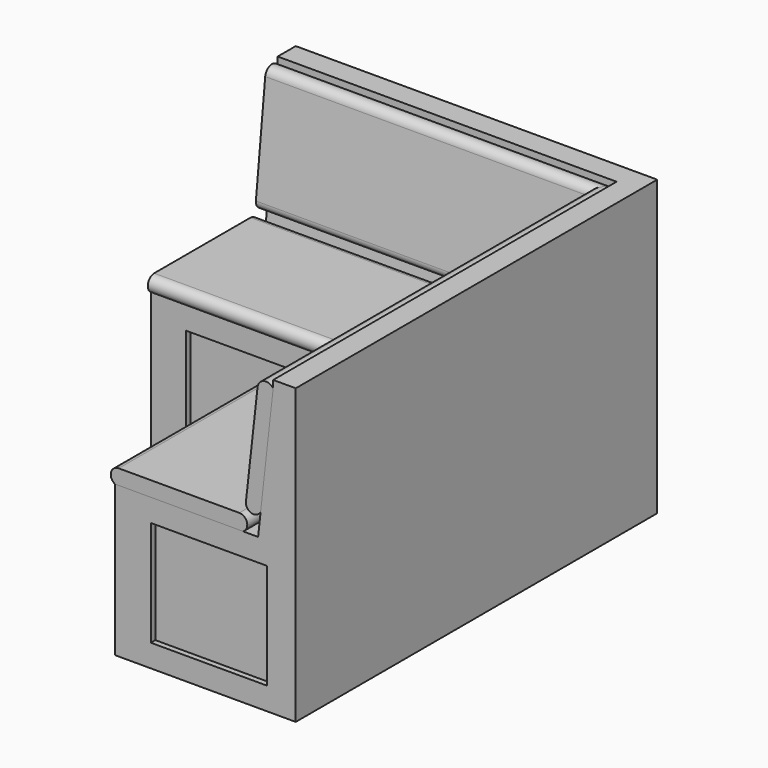
from build123d import *

# Parameters (mm, degrees)
F1_DEPTH  = 76.2
F2_DEPTH  = 25.4
F3_W      = 1168.4
F3_H      = 25.4
F4_DEPTH  = 889
F5_DEPTH  = 355.6
F7_DEPTH  = 76.2
F9_DEPTH  = 25.4
F11_DEPTH = 25.4
F13_DEPTH = 25.4
F14_DEPTH = 1193.8
F15_REACH = 1986.929480867
F16_W     = 406.1148560882
F16_H     = 381
F16_W_2   = 380.7148560882
F16_H_2   = 355.6
F17_DEPTH = 6.35
F18_W     = 435.2687171936
F18_H     = 381
F18_W_2   = 409.8687171936
F18_H_2   = 355.6
F19_DEPTH = 6.35
F20_W     = 742.6479629517
F20_H     = 381
F20_W_2   = 717.2479629517
F20_H_2   = 355.6
F21_DEPTH = 6.35
F22_W     = 417.8407884479
F22_H     = 381
F22_W_2   = 392.4407884479
F22_H_2   = 355.6
F23_DEPTH = 6.35
F25_DEPTH = 25.4
F26_DEPTH = 25.4
F28_REACH = 1987.1702785851
F30_REACH = 1682.3702785851
F32_DEPTH = 25.4


with BuildPart() as f1:
    # F0 (on Top) → F1 (new body)
    with BuildSketch(Plane.XY):
        Polygon((0, -1524), (0, 0), (-1219.2, 0), (-1219.2, -127), (-1219.2, -609.6), (-609.6, -609.6), (-609.6, -1524), (-127, -1524), align=None)
        Polygon((-584.2, -584.2), (-1193.8, -584.2), (-1193.8, -25.4), (-25.4, -25.4), (-25.4, -1498.6), (-584.2, -1498.6), align=None, mode=Mode.SUBTRACT)
    extrude(amount=F1_DEPTH)

    # F0 (on Top) → F2 (join)
    with BuildSketch(Plane.XY):
        Polygon((0, -1524), (0, 0), (-1219.2, 0), (-1219.2, -127), (-1219.2, -609.6), (-609.6, -609.6), (-609.6, -1524), (-127, -1524), align=None)
        Polygon((-584.2, -584.2), (-1193.8, -584.2), (-1193.8, -25.4), (-25.4, -25.4), (-25.4, -1498.6), (-584.2, -1498.6), align=None, mode=Mode.SUBTRACT)
        Polygon((-1193.8, -25.4), (-1193.8, -584.2), (-584.2, -584.2), (-584.2, -1498.6), (-25.4, -1498.6), (-25.4, -25.4), align=None)
    extrude(amount=F2_DEPTH)

    # F3 (on face) → F4 (join)
    with BuildSketch(Plane.XY.offset(76.2)):
        with Locations((-609.6, -12.7)):
            Rectangle(F3_W, F3_H)
        Polygon((-25.4, 0), (-25.4, -25.4), (-25.4, -1498.6), (0, -1498.6), (0, 0), align=None)
    extrude(amount=F4_DEPTH)

    # F3 (on face) → F5 (join)
    with BuildSketch(Plane.XY.offset(76.2)):
        Polygon((-1219.2, -479.6493053436), (-1219.2, -609.6), (-1102.1362543106, -609.6), (-1102.1362543106, -584.2), (-1193.8, -584.2), (-1193.8, -479.6493053436), align=None)
        Polygon((-1219.2, 0), (-1219.2, -98.9344492555), (-1193.8, -98.9344492555), (-1193.8, -25.4), (-1193.8, 0), align=None)
        Polygon((-692.267537117, -584.2), (-692.267537117, -609.6), (-609.6, -609.6), (-609.6, -683.7261915207), (-584.2, -683.7261915207), (-584.2, -584.2), align=None)
        Polygon((-584.2, -1400.9741544724), (-609.6, -1400.9741544724), (-609.6, -1524), (-488.8490438461, -1524), (-488.8490438461, -1498.6), (-584.2, -1498.6), align=None)
        Polygon((0, -1498.6), (-25.4, -1498.6), (-96.4082553983, -1498.6), (-96.4082553983, -1524), (0, -1524), align=None)
    extrude(amount=F5_DEPTH)

    # F6 (on face) → F7 (join)
    with BuildSketch(Plane.XY.offset(431.8)):
        Polygon((-692.267537117, -609.6), (-692.267537117, -584.2), (-1193.8, -584.2), (-1193.8, 0), (-1219.2, 0), (-1219.2, -609.6), align=None)
        Polygon((-584.2, -683.7261915207), (-584.2, -584.2), (-692.267537117, -584.2), (-692.267537117, -609.6), (-609.6, -609.6), (-609.6, -683.7261915207), align=None)
        Polygon((-584.2, -1498.6), (-584.2, -683.7261915207), (-609.6, -683.7261915207), (-609.6, -1524), (0, -1524), (0, -1498.6), align=None)
    extrude(amount=F7_DEPTH)

    # F8 (on face) → F9 (join)
    with BuildSketch(Plane.XZ.offset(1524)):
        Polygon((0, 508), (0, 965.2), (-54.3987713754, 965.2), (-105.1987713754, 508), align=None)
        Polygon((-105.1987713754, 508), (-54.3987713754, 965.2), (-76.2, 965.2), (-127, 508), align=None)
    extrude(amount=-F9_DEPTH)

    # F10 (on face) → F11 (join)
    with BuildSketch(Plane(origin=(-1219.2, 0, 0), x_dir=(0, -1, 0), z_dir=(-1, 0, 0))):
        Polygon((50.6436908324, 965.2), (0, 965.2), (0, 508), (101.4436908324, 508), align=None)
        Polygon((76.2, 965.2), (50.6436908324, 965.2), (101.4436908324, 508), (127, 508), align=None)
    extrude(amount=-F11_DEPTH)

    # F12 (on face) → F13 (join)
    with BuildSketch(Plane.XY.offset(508)):
        Polygon((-1193.8, 0), (-1193.8, -203.2), (-203.2, -203.2), (-203.2, -1498.6), (0, -1498.6), (0, 0), align=None)
    extrude(amount=-F13_DEPTH)

    # F10 (on face) → F14 (join, through all)
    with BuildSketch(Plane(origin=(-1219.2, 0, 0), x_dir=(0, -1, 0), z_dir=(-1, 0, 0))):
        Polygon((76.2, 965.2), (50.6436908324, 965.2), (101.4436908324, 508), (127, 508), align=None)
    extrude(amount=-F14_DEPTH)

    f15_end = f1.faces().sort_by_distance((-622.3, -101.6, 736.6))[0]
    # F8 (on face) → F15 (join, up to a face of the model that its end follows)
    with BuildSketch(Plane.XZ.offset(1524)):
        Polygon((-105.1987713754, 508), (-54.3987713754, 965.2), (-76.2, 965.2), (-127, 508), align=None)
    f15_long = extrude(amount=-F15_REACH, mode=Mode.PRIVATE)
    add(split(f15_long, bisect_by=f15_end, keep=Keep.TOP, mode=Mode.PRIVATE))

    # F31 (on face) → F32 (join)
    with BuildSketch(Plane.XY.offset(965.2)):
        Polygon((0, 0), (-1219.2, 0), (-1219.2, -76.2), (-76.2, -76.2), (-76.2, -1524), (0, -1524), align=None)
    extrude(amount=F32_DEPTH)


with BuildPart() as f17:
    # F16 (on face) → F17 (new body)
    with BuildSketch(Plane.YZ.offset(-1193.8)):
        with Locations((-289.2918772995, 254)):
            Rectangle(F16_W, F16_H)
        with Locations((-289.2918772995, 254)):
            Rectangle(F16_W_2, F16_H_2, mode=Mode.SUBTRACT)
        with Locations((-289.2918772995, 254)):
            Rectangle(F16_W_2, F16_H_2)
    extrude(amount=-F17_DEPTH)


with BuildPart() as f19:
    # F18 (on face) → F19 (new body)
    with BuildSketch(Plane(origin=(0, -584.2, 0), x_dir=(-1, 0, 0), z_dir=(0, 1, 0))):
        with Locations((897.2018957138, 254)):
            Rectangle(F18_W, F18_H)
        with Locations((897.2018957138, 254)):
            Rectangle(F18_W_2, F18_H_2, mode=Mode.SUBTRACT)
        with Locations((897.2018957138, 254)):
            Rectangle(F18_W_2, F18_H_2)
    extrude(amount=-F19_DEPTH)


with BuildPart() as f21:
    # F20 (on face) → F21 (new body)
    with BuildSketch(Plane.YZ.offset(-584.2)):
        with Locations((-1042.3501729965, 254)):
            Rectangle(F20_W, F20_H)
        with Locations((-1042.3501729965, 254)):
            Rectangle(F20_W_2, F20_H_2, mode=Mode.SUBTRACT)
        with Locations((-1042.3501729965, 254)):
            Rectangle(F20_W_2, F20_H_2)
    extrude(amount=-F21_DEPTH)


with BuildPart() as f23:
    # F22 (on face) → F23 (new body)
    with BuildSketch(Plane(origin=(0, -1498.6, 0), x_dir=(-1, 0, 0), z_dir=(0, 1, 0))):
        with Locations((292.6286496222, 254)):
            Rectangle(F22_W, F22_H)
        with Locations((292.6286496222, 254)):
            Rectangle(F22_W_2, F22_H_2, mode=Mode.SUBTRACT)
        with Locations((292.6286496222, 254)):
            Rectangle(F22_W_2, F22_H_2)
    extrude(amount=-F23_DEPTH)


with BuildPart() as f25:
    # F24 (on face) → F25 (new body)
    with BuildSketch(Plane.XY.offset(508)):
        Polygon((-203.2, -203.2), (-1193.8, -203.2), (-1193.8, -584.2), (-584.2, -584.2), align=None)
    extrude(amount=-F25_DEPTH)


with BuildPart() as f26:
    # F24 (on face) → F26 (new body)
    with BuildSketch(Plane.XY.offset(508)):
        Polygon((-203.2, -1498.6), (-203.2, -203.2), (-584.2, -584.2), (-584.2, -1498.6), align=None)
    extrude(amount=-F26_DEPTH)


with BuildPart() as f28:
    f28_end = Plane(origin=(-393.7, -393.7, 495.3), x_dir=(-0.7071067812, -0.7071067812, 0), z_dir=(0.7071067812, -0.7071067812, 0))
    # F27 (on face) → F28 (new body, up to a plane its end follows)
    with BuildSketch(Plane.XZ.offset(1524)):
        with BuildLine():
            ThreePointArc((-596.9, 558.8), (-623.0817207227, 538.3579301807), (-609.6, 508))
            Line((-609.6, 508), (-177.8, 508))
            ThreePointArc((-177.8, 508), (-164.3182792773, 538.3579301807), (-190.5, 558.8))
            Line((-190.5, 558.8), (-596.9, 558.8))
        make_face()
    f28_long = extrude(amount=-F28_REACH, mode=Mode.PRIVATE)
    add(split(f28_long, bisect_by=f28_end, keep=Keep.TOP, mode=Mode.PRIVATE))


with BuildPart() as f28b:
    f28_2_end = Plane(origin=(-393.7, -393.7, 495.3), x_dir=(-0.7071067812, -0.7071067812, 0), z_dir=(0.7071067812, -0.7071067812, 0))
    # F27 (on face) → F28, piece 2 (new body, up to a plane its end follows)
    with BuildSketch(Plane.XZ.offset(1524)):
        with BuildLine():
            ThreePointArc((-167.9931801186, 599.0749439501), (-148.6035006779, 571.1242906487), (-118.2744114345, 586.5302970894))
            Line((-118.2744114345, 586.5302970894), (-76.2, 965.2))
            ThreePointArc((-76.2, 965.2), (-106.9137050785, 977.2615951465), (-128.7237294464, 952.5))
            Line((-128.7237294464, 952.5), (-167.9931801186, 599.0749439501))
        make_face()
    f28_2_long = extrude(amount=-F28_REACH, mode=Mode.PRIVATE)
    add(split(f28_2_long, bisect_by=f28_2_end, keep=Keep.TOP, mode=Mode.PRIVATE))


with BuildPart() as f30:
    f30_end = Plane(origin=(-393.7, -393.7, 495.3), x_dir=(0.7071067812, 0.7071067812, 0), z_dir=(-0.7071067812, 0.7071067812, 0))
    # F29 (on face) → F30 (new body, up to a plane its end follows)
    with BuildSketch(Plane(origin=(-1219.2, 0, 0), x_dir=(0, -1, 0), z_dir=(-1, 0, 0))):
        with BuildLine():
            Line((177.8, 508), (609.6, 508))
            ThreePointArc((609.6, 508), (623.0817207227, 538.3579301807), (596.9, 558.8))
            Line((596.9, 558.8), (190.5, 558.8))
            ThreePointArc((190.5, 558.8), (164.3182792773, 538.3579301807), (177.8, 508))
        make_face()
    f30_long = extrude(amount=-F30_REACH, mode=Mode.PRIVATE)
    add(split(f30_long, bisect_by=f30_end, keep=Keep.TOP, mode=Mode.PRIVATE))


with BuildPart() as f30b:
    f30_2_end = Plane(origin=(-393.7, -393.7, 495.3), x_dir=(0.7071067812, 0.7071067812, 0), z_dir=(-0.7071067812, 0.7071067812, 0))
    # F29 (on face) → F30, piece 2 (new body, up to a plane its end follows)
    with BuildSketch(Plane(origin=(-1219.2, 0, 0), x_dir=(0, -1, 0), z_dir=(-1, 0, 0))):
        with BuildLine():
            Line((76.2, 965.2), (118.2744114345, 586.5302970894))
            ThreePointArc((118.2744114345, 586.5302970894), (148.6035006779, 571.1242906487), (167.9931801186, 599.0749439501))
            Line((167.9931801186, 599.0749439501), (128.7237294464, 952.5))
            ThreePointArc((128.7237294464, 952.5), (106.9137050785, 977.2615951465), (76.2, 965.2))
        make_face()
    f30_2_long = extrude(amount=-F30_REACH, mode=Mode.PRIVATE)
    add(split(f30_2_long, bisect_by=f30_2_end, keep=Keep.TOP, mode=Mode.PRIVATE))


solid = Compound([f1.part, f17.part, f19.part, f21.part, f23.part, f25.part, f26.part, f28.part, f28b.part, f30.part, f30b.part])
